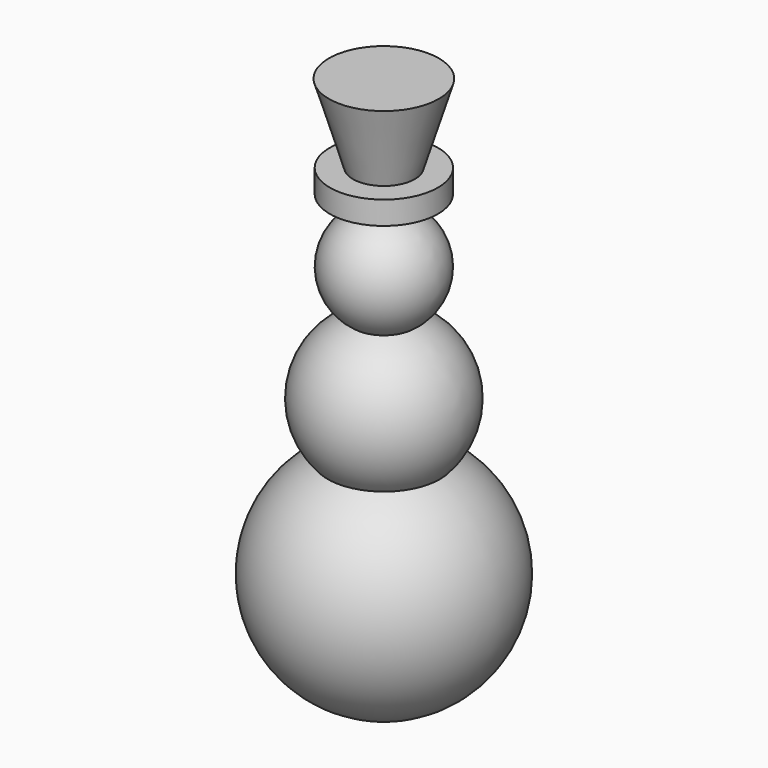
from build123d import *


# Not quite as in the source:
# - a feature names something its author has since deleted; it is built from what else it names


with BuildPart() as f1:
    # F0 (on Front) → F1 (revolve)
    with BuildSketch(Plane.XZ):
        with BuildLine():
            Line((0, 0), (0, -38.1))
            ThreePointArc((0, -38.1), (36.8901663726, -9.525), (18.4450831863, 33.3375))
            ThreePointArc((18.4450831863, 33.3375), (24.8680463142, 55.9710997394), (9.9547263147, 74.168))
            ThreePointArc((9.9547263147, 74.168), (17.7294771599, 90.2394176477), (7.6284402255, 104.9603642464))
            ThreePointArc((7.6284402255, 104.9603642464), (12.0633962281, 108.7560954443), (17.78, 109.9379801202))
            Line((17.78, 109.9379801202), (17.78, 117.5579801202))
            Line((17.78, 117.5579801202), (10.1936982811, 117.5579801202))
            Line((10.1936982811, 117.5579801202), (18.0881139505, 143.3620005846))
            Line((18.0881139505, 143.3620005846), (0, 143.3620005846))
            Line((0, 143.3620005846), (0, 0))
        make_face()
    revolve(axis=Axis((0, 0, 71.6810002923), (0, 0, -1)))


solid = f1.part
